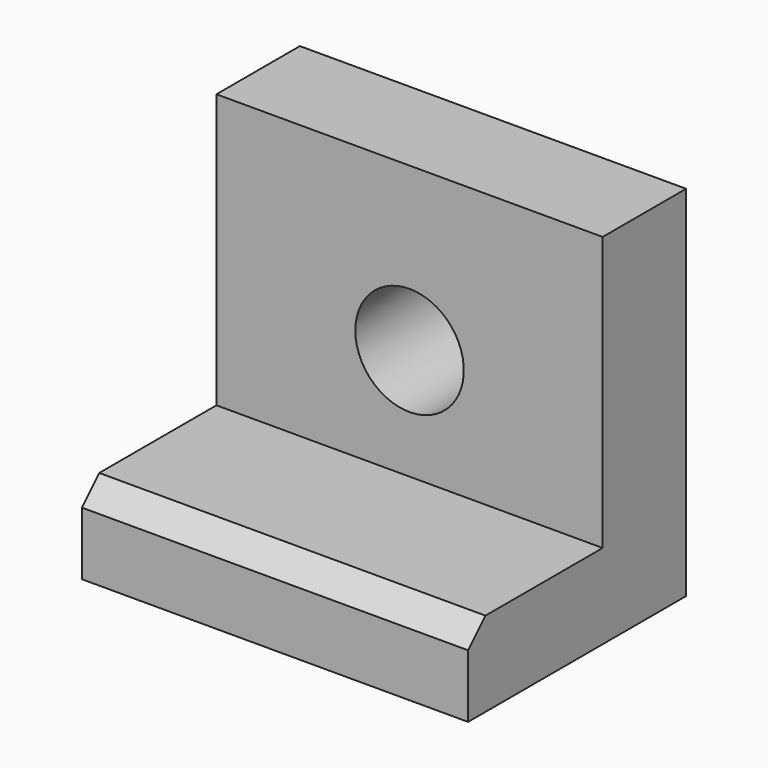
from build123d import *

# Parameters (mm, degrees)
F1_DEPTH = 45.212
F2_R     = 12.7
F3_DEPTH = 25.4
F4_SIZE  = 5.08


# Not quite as in the source:
# - a feature of the source that left no trace in its solid (it failed there, or was rolled back) is left out


with BuildPart() as f1:
    # F0 (on Right) → F1 (new body, symmetric)
    with BuildSketch(Plane.YZ):
        Polygon((24.4213882834, -39.0742197633), (24.4213882834, 44.8742993176), (0, 44.8742993176), (0, -19.2318409681), (-39.3794849515, -19.2318409681), (-39.3794849515, -39.0742197633), align=None)
    extrude(amount=F1_DEPTH, both=True)

    # F2 (on face) → F3 (cut)
    with BuildSketch(Plane(origin=(0, 24.4213882834, 0), x_dir=(-1, 0, 0), z_dir=(0, 1, 0))):
        with Locations((0, 6.7742993176)):
            Circle(F2_R)
    extrude(amount=-F3_DEPTH, mode=Mode.SUBTRACT)

    # F4
    f4_edges = [f1.edges().sort_by_distance(p)[0] for p in [
        (0, -39.379485, -19.231841),
    ]]
    chamfer(f4_edges, length=F4_SIZE)


solid = f1.part
